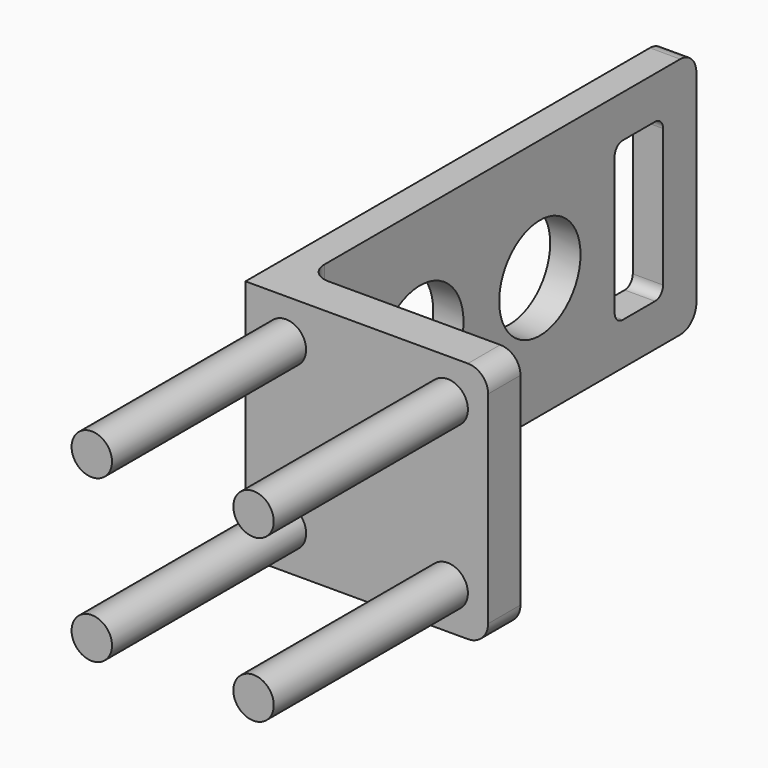
from build123d import *

# Parameters (mm, degrees)
F0_W      = 304.8
F0_H      = 304.8
F1_DEPTH  = 50.8
F2_R      = 25.4
F3_DEPTH  = 304.8
F6_W      = 38.1
F6_H      = 304.8
F7_DEPTH  = 609.6
F8_R      = 25.4
F9_R      = 25.4
F10_R     = 25.4
F11_R     = 68.2122039911
F12_DEPTH = 38.1
F13_R     = 63.8417796902
F14_DEPTH = 38.1
F15_W     = 76.0798454285
F15_H     = 198.4691917896
F16_DEPTH = 38.1
F17_R     = 12.7


with BuildPart() as f1:
    # F0 (on Front) → F1 (new body)
    with BuildSketch(Plane.XZ):
        Rectangle(F0_W, F0_H)
    extrude(amount=F1_DEPTH)

    # F2 (on face) → F3 (join)
    with BuildSketch(Plane.XZ.offset(50.8)):
        with Locations((-101.6, 101.6)):
            Circle(F2_R)
    extrude(amount=F3_DEPTH)


with BuildPart() as f4_1:
    # F4: instance of F1
    add(f1.part.mirror(Plane.XY))


with BuildPart() as f1_1:
    add(f1.part)

    add(f4_1.part)  # F5 merges F4_1
    # F5: F1, F4_1 across plane
    add(f1.part.mirror(Plane.YZ))
    add(f4_1.part.mirror(Plane.YZ))

    # F6 (on face) → F7 (join)
    with BuildSketch(Plane(origin=(0, 0, 0), x_dir=(-1, 0, 0), z_dir=(0, 1, 0))):
        with Locations((133.35, 0)):
            Rectangle(F6_W, F6_H)
    extrude(amount=F7_DEPTH)

    # F8
    f8_edges = [f1_1.edges().sort_by_distance(p)[0] for p in [
        (-133.35, 609.6, 152.4),
        (-133.35, 609.6, -152.4),
    ]]
    fillet(f8_edges, radius=F8_R)

    # F9
    f9_edges = [f1_1.edges().sort_by_distance(p)[0] for p in [
        (-114.3, 0, 0),
        (152.4, -25.4, 152.4),
    ]]
    fillet(f9_edges, radius=F9_R)

    # F10
    f10_edges = [f1_1.edges().sort_by_distance(p)[0] for p in [
        (152.4, -25.4, -152.4),
    ]]
    fillet(f10_edges, radius=F10_R)

    # F11 (on face) → F12 (cut, through all)
    with BuildSketch(Plane.YZ.offset(-114.3)):
        with Locations((175.7188588381, 0)):
            Circle(F11_R)
    extrude(amount=-F12_DEPTH, mode=Mode.SUBTRACT)

    # F13 (on face) → F14 (cut, through all)
    with BuildSketch(Plane.YZ.offset(-114.3)):
        with Locations((363.809466362, 0)):
            Circle(F13_R)
    extrude(amount=-F14_DEPTH, mode=Mode.SUBTRACT)

    # F15 (on face) → F16 (cut, through all)
    with BuildSketch(Plane.YZ.offset(-114.3)):
        with Locations((519.2769765854, 0)):
            Rectangle(F15_W, F15_H)
    extrude(amount=-F16_DEPTH, mode=Mode.SUBTRACT)

    # F17
    f17_edges = [f1_1.edges().sort_by_distance(p)[0] for p in [
        (-133.35, 557.316899, -99.234596),
        (-133.35, 557.316899, 99.234596),
        (-133.35, 481.237054, 99.234596),
        (-133.35, 481.237054, -99.234596),
    ]]
    fillet(f17_edges, radius=F17_R)


solid = f1_1.part
